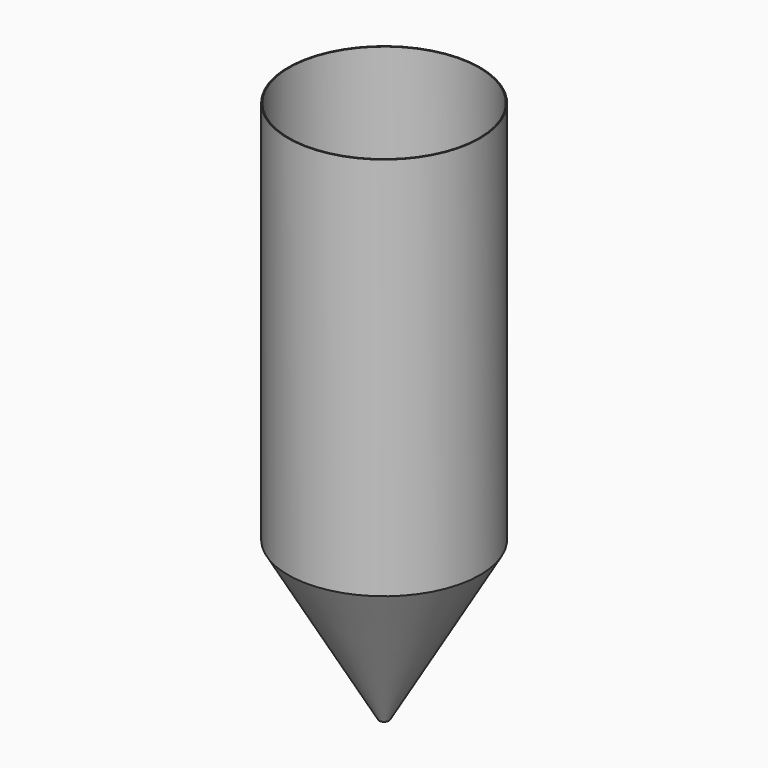
from build123d import *

# Parameters (mm, degrees)
F0_R     = 250
F1_DEPTH = 1000
F2_R     = 250
F4_T     = -2.5
F5_R     = 12.5
F6_DEPTH = 433.0137019922


# Not quite as in the source:
# - an extrude whose draft closes it to a point is written as a loft to that point


with BuildPart() as f1:
    # F0 (on Top) → F1 (new body)
    with BuildSketch(Plane.XY):
        Circle(F0_R)
    extrude(amount=F1_DEPTH)

    # F2 (on face) → F3 section 0
    with BuildSketch(Plane(origin=(0, 0, 0), x_dir=(1, 0, 0), z_dir=(0, 0, -1)), mode=Mode.PRIVATE) as f3_s0:
        Circle(F2_R)
    loft([f3_s0.sketch, Vertex(0, 0, -433.0127018922)], ruled=True)

    # F4
    f4_openings = [f1.faces().sort_by_distance(p)[0] for p in [
        (0, 0, 1000),
    ]]
    offset(amount=F4_T, openings=f4_openings)

    # F5 (on Top) → F6 (cut, through all)
    with BuildSketch(Plane.XY):
        Circle(F5_R)
    extrude(amount=-F6_DEPTH, mode=Mode.SUBTRACT)


solid = f1.part
